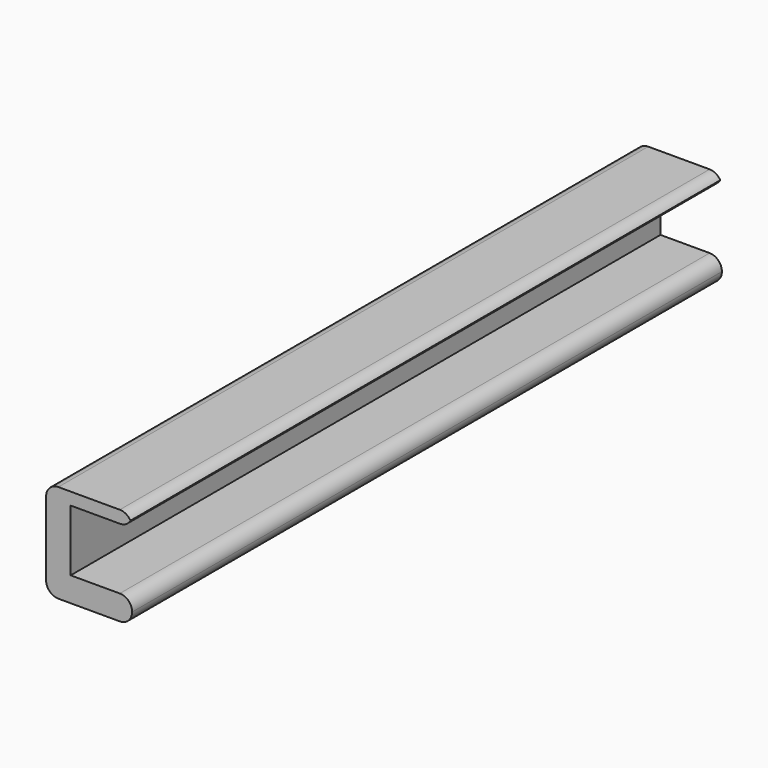
from build123d import *

# Parameters (mm, degrees)
F0_W        = 6.35
F0_H        = 2.54
F1_DEPTH    = 76.2
F2_R        = 1.27
F3_T1_DEPTH = 82.55


# Not quite as in the source:
# - a fillet or chamfer that OpenCascade refuses, or shapes differently, is made with other operations: its cross-section is extruded or revolved along the edge and cut away or added


with BuildPart() as f1:
    # F0 (on Front) → F1 (new body)
    with BuildSketch(Plane.XZ):
        Polygon((-43.1055540526, 26.5985474133), (-40.5655540526, 26.5985474133), (-34.2155540526, 26.5985474133), (-34.2155540526, 27.8685474133), (-43.1055540526, 27.8685474133), align=None)
        Polygon((-40.5655540526, 20.2485474133), (-40.5655540526, 26.5985474133), (-43.1055540526, 26.5985474133), (-43.1055540526, 17.7085474133), (-40.5655540526, 17.7085474133), align=None)
        with Locations((-37.3905540526, 18.9785474133)):
            Rectangle(F0_W, F0_H)
    extrude(amount=F1_DEPTH)

    # F2
    f2_edges = [f1.edges().sort_by_distance(p)[0] for p in [
        (-43.105554, -38.1, 27.868547),
    ]]
    fillet(f2_edges, radius=F2_R)

    # F3: fillet of radius 1.27 on 5 edges, made by hand

    # F3_s2 → F3_t1 (cut)
    with BuildSketch(Plane.XZ.offset(-3.175)):
        with BuildLine():
            ThreePointArc((-43.1055540526, 18.9785474133), (-42.7335796647, 18.0805218012), (-41.8355540526, 17.7085474133))
            Line((-41.8355540526, 17.7085474133), (-43.1055540526, 17.7085474133))
            Line((-43.1055540526, 17.7085474133), (-43.1055540526, 18.9785474133))
        make_face()
        with BuildLine():
            ThreePointArc((-34.2155540526, 27.8685474133), (-34.5875284405, 26.9705218012), (-35.4855540526, 26.5985474133))
            Line((-35.4855540526, 26.5985474133), (-34.2155540526, 26.5985474133))
            Line((-34.2155540526, 26.5985474133), (-34.2155540526, 27.8685474133))
        make_face()
        with BuildLine():
            ThreePointArc((-34.2155540526, 18.9785474133), (-34.5875284405, 19.8765730255), (-35.4855540526, 20.2485474133))
            Line((-35.4855540526, 20.2485474133), (-34.2155540526, 20.2485474133))
            Line((-34.2155540526, 20.2485474133), (-34.2155540526, 18.9785474133))
        make_face()
        with BuildLine():
            ThreePointArc((-35.4855540526, 17.7085474133), (-34.5875284405, 18.0805218012), (-34.2155540526, 18.9785474133))
            Line((-34.2155540526, 18.9785474133), (-34.2155540526, 17.7085474133))
            Line((-34.2155540526, 17.7085474133), (-35.4855540526, 17.7085474133))
        make_face()
        with BuildLine():
            ThreePointArc((-35.4855540526, 27.8685474133), (-34.5875284405, 27.4965730255), (-34.2155540526, 26.5985474133))
            Line((-34.2155540526, 26.5985474133), (-34.2155540526, 27.8685474133))
            Line((-34.2155540526, 27.8685474133), (-35.4855540526, 27.8685474133))
        make_face()
    extrude(amount=F3_T1_DEPTH, mode=Mode.SUBTRACT)


solid = f1.part
